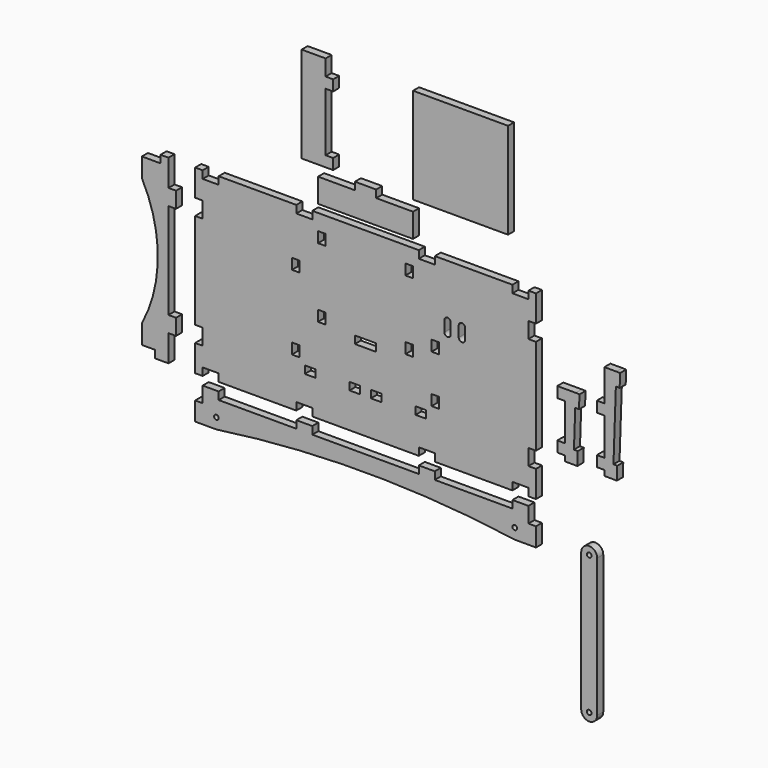
from build123d import *

# Parameters (mm, degrees)
F1_W     = 18.034
F1_H     = 25.4
F2_DEPTH = 18.034
F1_W_2   = 50.8
F1_H_2   = 18.034
F1_W_3   = 25.4
F1_H_3   = 38.1
F1_W_4   = 38.1
F1_R     = 5.55625
F1_W_5   = 226.568
F1_H_4   = 228.6


# Not quite as in the source:
# - a variable given as a bare number and used for a length is read in inches; the dataset says mm whatever the document's units were


with BuildPart() as f2:
    # F1 (on Front) → F2 (new body)
    with BuildSketch(Plane.XZ):
        Polygon((-152.4, 317.5), (-95.25, 317.5), (-95.25, 342.9), (-95.25, 482.6), (-95.25, 508), (-95.25, 546.1), (-152.4, 546.1), align=None)
        with Locations((-86.233, 495.3)):
            Rectangle(F1_W, F1_H)
        with Locations((-86.233, 330.2)):
            Rectangle(F1_W, F1_H)
    extrude(amount=F2_DEPTH)


with BuildPart() as f2b:
    # F1 (on Front) → F2, piece 2 (new body)
    with BuildSketch(Plane.XZ):
        with Locations((0, 301.117)):
            Rectangle(F1_W_2, F1_H_2)
        Polygon((-113.284, 292.1), (-113.284, 234.95), (113.284, 234.95), (113.284, 292.1), (25.4, 292.1), (-25.4, 292.1), align=None)
    extrude(amount=F2_DEPTH)


with BuildPart() as f2c:
    # F1 (on Front) → F2, piece 3 (new body)
    with BuildSketch(Plane.XZ):
        Polygon((-388.366, 215.9), (-406.4, 215.9), (-406.4, 152.4), (-388.366, 152.4), (-388.366, 114.3), (-406.4, 114.3), (-406.4, -114.3), (-388.366, -114.3), (-388.366, -152.4), (-406.4, -152.4), (-406.4, -215.9), (-388.366, -215.9), (-388.366, -197.866), (-350.266, -197.866), (-350.266, -215.9), (-165.1, -215.9), (-165.1, -197.866), (-127, -197.866), (-127, -215.9), (127, -215.9), (127, -197.866), (165.1, -197.866), (165.1, -215.9), (350.266, -215.9), (350.266, -197.866), (388.366, -197.866), (388.366, -215.9), (406.4, -215.9), (406.4, -152.4), (388.366, -152.4), (388.366, -114.3), (406.4, -114.3), (406.4, 114.3), (388.366, 114.3), (388.366, 152.4), (406.4, 152.4), (406.4, 215.9), (388.366, 215.9), (388.366, 197.866), (350.266, 197.866), (350.266, 215.9), (165.1, 215.9), (165.1, 197.866), (127, 197.866), (127, 215.9), (-127, 215.9), (-127, 197.866), (-165.1, 197.866), (-165.1, 215.9), (-350.266, 215.9), (-350.266, 197.866), (-388.366, 197.866), align=None)
        with Locations((-132.08, -123.317)):
            Rectangle(F1_W_3, F1_H_2, mode=Mode.SUBTRACT)
        with Locations((-166.497, -88.9)):
            Rectangle(F1_W, F1_H, mode=Mode.SUBTRACT)
        with Locations((-25.4, -123.317)):
            Rectangle(F1_W_3, F1_H_2, mode=Mode.SUBTRACT)
        with Locations((25.4, -123.317)):
            Rectangle(F1_W_3, F1_H_2, mode=Mode.SUBTRACT)
        with Locations((132.08, -123.317)):
            Rectangle(F1_W_3, F1_H_2, mode=Mode.SUBTRACT)
        with Locations((166.497, -88.9)):
            Rectangle(F1_W, F1_H, mode=Mode.SUBTRACT)
        with Locations((-166.497, 88.9)):
            Rectangle(F1_W, F1_H, mode=Mode.SUBTRACT)
        with Locations((-104.267, 0)):
            Rectangle(F1_W, F1_H, mode=Mode.SUBTRACT)
        with Locations((0, -21.717)):
            Rectangle(F1_W_2, F1_H_2, mode=Mode.SUBTRACT)
        with Locations((-104.267, 165.1)):
            Rectangle(F1_W, F1_H, mode=Mode.SUBTRACT)
        with Locations((104.267, 0)):
            Rectangle(F1_W, F1_H, mode=Mode.SUBTRACT)
        with Locations((166.497, 25.4)):
            Rectangle(F1_W, F1_H, mode=Mode.SUBTRACT)
        with BuildLine():
            Line((187.96, 63.5), (187.96, 88.9))
            ThreePointArc((187.96, 88.9), (195.58, 96.52), (203.2, 88.9))
            Line((203.2, 88.9), (203.2, 63.5))
            ThreePointArc((203.2, 63.5), (195.58, 55.88), (187.96, 63.5))
        make_face(mode=Mode.SUBTRACT)
        with BuildLine():
            Line((222.25, 63.5), (222.25, 88.9))
            ThreePointArc((222.25, 88.9), (229.87, 96.52), (237.49, 88.9))
            Line((237.49, 88.9), (237.49, 63.5))
            ThreePointArc((237.49, 63.5), (229.87, 55.88), (222.25, 63.5))
        make_face(mode=Mode.SUBTRACT)
        with Locations((104.267, 165.1)):
            Rectangle(F1_W, F1_H, mode=Mode.SUBTRACT)
    extrude(amount=F2_DEPTH)


with BuildPart() as f2d:
    # F1 (on Front) → F2, piece 4 (new body)
    with BuildSketch(Plane.XZ):
        with BuildLine():
            Line((-469.9, 215.9), (-488.95, 215.9))
            Line((-488.95, 215.9), (-488.95, 197.866))
            Line((-488.95, 197.866), (-533.4, 197.866))
            Line((-533.4, 197.866), (-533.4, 152.4))
            ThreePointArc((-533.4, 152.4), (-495.3, 0), (-533.4, -152.4))
            Line((-533.4, -152.4), (-533.4, -197.866))
            Line((-533.4, -197.866), (-501.65, -197.866))
            Line((-501.65, -197.866), (-501.65, -215.9))
            Line((-501.65, -215.9), (-469.9, -215.9))
            Line((-469.9, -215.9), (-469.9, -152.4))
            Line((-469.9, -152.4), (-469.9, -114.3))
            Line((-469.9, -114.3), (-469.9, 114.3))
            Line((-469.9, 114.3), (-469.9, 152.4))
            Line((-469.9, 152.4), (-469.9, 215.9))
        make_face()
        with Locations((-460.883, 133.35)):
            Rectangle(F1_W, F1_H_3)
        with Locations((-460.883, -133.35)):
            Rectangle(F1_W, F1_H_3)
    extrude(amount=F2_DEPTH)


with BuildPart() as f2e:
    # F1 (on Front) → F2, piece 5 (new body)
    with BuildSketch(Plane.XZ):
        with Locations((466.217, 25.4)):
            Rectangle(F1_W, F1_H)
        Polygon((475.234, 12.7), (475.234, -76.2), (475.234, -101.6), (475.234, -114.3), (495.8715, -114.3), (496.9732665927, -82.5691221304), (500.061400074, 6.3691221304), (501.1631666667, 38.1), (475.234, 38.1), align=None)
        Polygon((510.1747359816, 37.7870982877), (501.1631666667, 38.1), (500.061400074, 6.3691221304), (509.0729693889, 6.0562204181), align=None)
        Polygon((496.9732665927, -82.5691221304), (495.8715, -114.3), (504.883069315, -114.6129017123), (505.9848359077, -82.8820238427), align=None)
        with Locations((466.217, -88.9)):
            Rectangle(F1_W, F1_H)
    extrude(amount=F2_DEPTH)


with BuildPart() as f2f:
    # F1 (on Front) → F2, piece 6 (new body)
    with BuildSketch(Plane.XZ):
        with Locations((560.451, -88.9)):
            Rectangle(F1_W, F1_H)
        with Locations((560.451, 25.4)):
            Rectangle(F1_W, F1_H)
        Polygon((607.054569315, 113.9870982877), (598.043, 114.3), (596.9412334073, 82.5691221304), (605.9528027223, 82.2562204181), align=None)
        Polygon((600.2188359077, -82.8820238427), (591.2072665927, -82.5691221304), (590.1055, -114.3), (599.117069315, -114.6129017123), align=None)
        Polygon((569.468, 114.3), (569.468, 38.1), (569.468, 12.7), (569.468, -76.2), (569.468, -101.6), (569.468, -114.3), (590.1055, -114.3), (591.2072665927, -82.5691221304), (596.9412334073, 82.5691221304), (598.043, 114.3), align=None)
    extrude(amount=F2_DEPTH)


with BuildPart() as f2g:
    # F1 (on Front) → F2, piece 7 (new body)
    with BuildSketch(Plane.XZ):
        with Locations((-369.316, -244.983)):
            Rectangle(F1_W_4, F1_H_2)
        with BuildLine():
            Line((-350.266, -254), (-388.366, -254))
            Line((-388.366, -254), (-388.366, -273.05))
            Line((-388.366, -273.05), (-406.4, -273.05))
            Line((-406.4, -273.05), (-406.4, -317.5))
            Line((-406.4, -317.5), (-355.6, -317.5))
            ThreePointArc((-355.6, -317.5), (-6.4933112155, -292.1084262284), (342.7404742076, -315.6875545364))
            Line((342.7404742075, -315.6875545364), (337.3404342206, -297.5305393424))
            ThreePointArc((337.3404342206, -297.5305393424), (350.1694606576, -273.8404342206), (373.8595657794, -286.6694606576))
            Line((373.8595657794, -286.6694606576), (383.0288121278, -317.5))
            Line((383.0288121278, -317.5), (406.4, -317.5))
            Line((406.4, -317.5), (406.4, -273.05))
            Line((406.4, -273.05), (388.366, -273.05))
            Line((388.366, -273.05), (388.366, -254))
            Line((388.366, -254), (350.266, -254))
            Line((350.266, -254), (165.1, -254))
            Line((165.1, -254), (127, -254))
            Line((127, -254), (-127, -254))
            Line((-127, -254), (-165.1, -254))
            Line((-165.1, -254), (-350.266, -254))
        make_face()
        with Locations((-355.6, -292.1)):
            Circle(F1_R, mode=Mode.SUBTRACT)
        with Locations((-146.05, -244.983)):
            Rectangle(F1_W_4, F1_H_2)
        with Locations((146.05, -244.983)):
            Rectangle(F1_W_4, F1_H_2)
        with Locations((369.316, -244.983)):
            Rectangle(F1_W_4, F1_H_2)
        with BuildLine():
            Line((337.3404342206, -297.5305393424), (342.7404742075, -315.6875545364))
            ThreePointArc((342.7404742076, -315.6875545364), (349.1714130893, -316.5854335051), (355.6, -317.5))
            Line((355.6, -317.5), (383.0288121278, -317.5))
            Line((383.0288121278, -317.5), (373.8595657794, -286.6694606576))
            ThreePointArc((373.8595657794, -286.6694606576), (374.4513557615, -289.3561184516), (374.65, -292.1))
            ThreePointArc((374.65, -292.1), (358.3438815484, -310.9513557615), (337.3404342206, -297.5305393424))
        make_face()
        with BuildLine():
            Line((350.2742933144, -293.6839073082), (337.3404342206, -297.5305393424))
            ThreePointArc((337.3404342206, -297.5305393424), (358.3438815484, -310.9513557615), (374.65, -292.1))
            ThreePointArc((374.65, -292.1), (374.4513557615, -289.3561184516), (373.8595657794, -286.6694606576))
            Line((373.8595657794, -286.6694606576), (360.9257066856, -290.5160926918))
            ThreePointArc((360.9257066856, -290.5160926918), (361.0983120971, -291.2997012151), (361.15625, -292.1))
            ThreePointArc((361.15625, -292.1), (356.4002987849, -297.5983120971), (350.2742933144, -293.6839073082))
        make_face()
        with BuildLine():
            ThreePointArc((373.8595657794, -286.6694606576), (350.1694606576, -273.8404342206), (337.3404342206, -297.5305393424))
            Line((337.3404342206, -297.5305393424), (350.2742933144, -293.6839073082))
            ThreePointArc((350.2742933144, -293.6839073082), (354.0160926918, -286.7742933144), (360.9257066856, -290.5160926918))
            Line((360.9257066856, -290.5160926918), (373.8595657794, -286.6694606576))
        make_face()
    extrude(amount=F2_DEPTH)


with BuildPart() as f2h:
    # F1 (on Front) → F2, piece 8 (new body)
    with BuildSketch(Plane.XZ):
        with BuildLine():
            Line((552.45, -622.3), (552.45, -292.1))
            ThreePointArc((552.45, -292.1), (533.4, -273.05), (514.35, -292.1))
            Line((514.35, -292.1), (514.35, -622.3))
            ThreePointArc((514.35, -622.3), (533.4, -641.35), (552.45, -622.3))
        make_face()
        with Locations((533.4, -622.3)):
            Circle(F1_R, mode=Mode.SUBTRACT)
        with Locations((533.4, -292.1)):
            Circle(F1_R, mode=Mode.SUBTRACT)
    extrude(amount=F2_DEPTH)


with BuildPart() as f2i:
    # F1 (on Front) → F2, piece 9 (new body)
    with BuildSketch(Plane.XZ):
        with Locations((226.568, 431.8)):
            Rectangle(F1_W_5, F1_H_4)
    extrude(amount=F2_DEPTH)


solid = Compound([f2.part, f2b.part, f2c.part, f2d.part, f2e.part, f2f.part, f2g.part, f2h.part, f2i.part])
